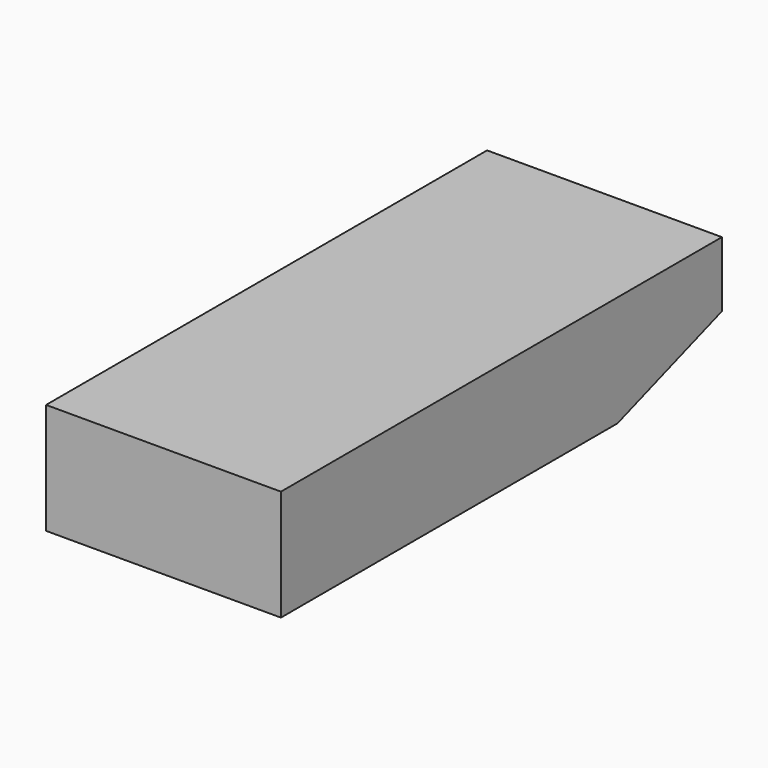
from build123d import *

# Parameters (mm, degrees)
F0_W     = 914.4
F0_H     = 431.8
F1_DEPTH = 1073.15
F3_DEPTH = 914.401


# Not quite as in the source:
# - a feature names something its author has since deleted; it is built from what else it names


with BuildPart() as f1:
    # F0 (on Front) → F1 (new body, symmetric)
    with BuildSketch(Plane.XZ):
        Rectangle(F0_W, F0_H)
    extrude(amount=F1_DEPTH, both=True)

    # F2 (on face) → F3 (cut, through all)
    with BuildSketch(Plane.YZ.offset(457.2)):
        Polygon((1073.15, -215.9), (1073.15, -38.1), (565.15, -215.9), align=None)
    extrude(amount=-F3_DEPTH, mode=Mode.SUBTRACT)


solid = f1.part
